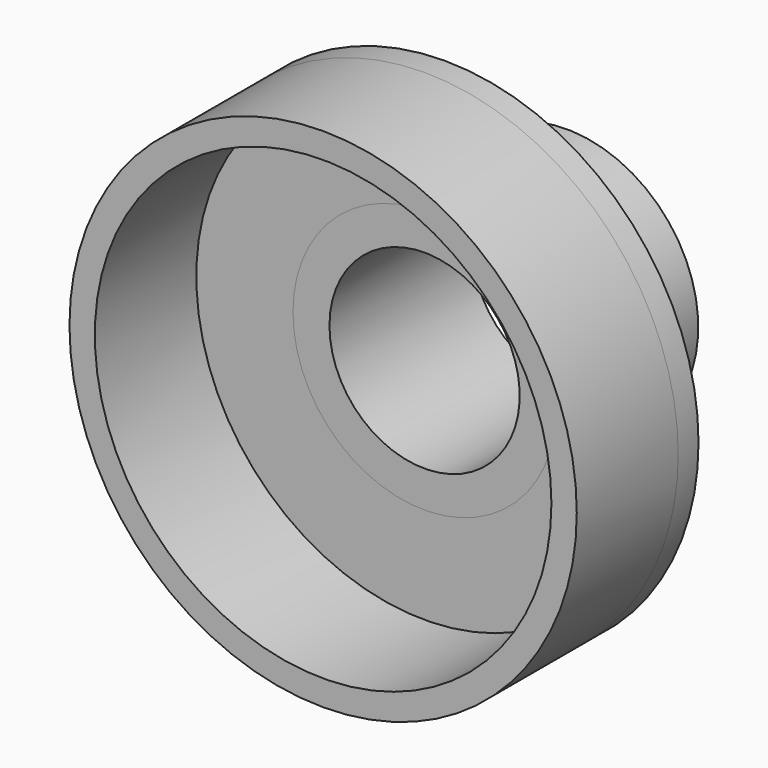
from build123d import *

# Parameters (mm, degrees)
F0_R     = 25.4
F0_R_2   = 22.86
F1_DEPTH = 3.81
F2_DEPTH = 12.7
F3_R     = 25.4
F3_R_2   = 22.86
F3_R_3   = 13.1826
F4_DEPTH = 2.54
F3_R_4   = 9.525
F5_DEPTH = 17.78


with BuildPart() as f1:
    # F0 (on Front) → F1 (new body)
    with BuildSketch(Plane.XZ):
        Circle(F0_R)
        Circle(F0_R_2, mode=Mode.SUBTRACT)
    extrude(amount=F1_DEPTH)

    # F0 (on Front) → F2 (join)
    with BuildSketch(Plane.XZ):
        Circle(F0_R)
        Circle(F0_R_2, mode=Mode.SUBTRACT)
    extrude(amount=F2_DEPTH)

    # F3 (on face) → F4 (join)
    with BuildSketch(Plane(origin=(0, 0, 0), x_dir=(-1, 0, 0), z_dir=(0, 1, 0))):
        Circle(F3_R)
        Circle(F3_R_2, mode=Mode.SUBTRACT)
        Circle(F3_R_2)
        Circle(F3_R_3, mode=Mode.SUBTRACT)
    extrude(amount=F4_DEPTH)

    # F3 (on face) → F5 (join)
    with BuildSketch(Plane(origin=(0, 0, 0), x_dir=(-1, 0, 0), z_dir=(0, 1, 0))):
        Circle(F3_R_3)
        Circle(F3_R_4, mode=Mode.SUBTRACT)
    extrude(amount=F5_DEPTH)


solid = f1.part
